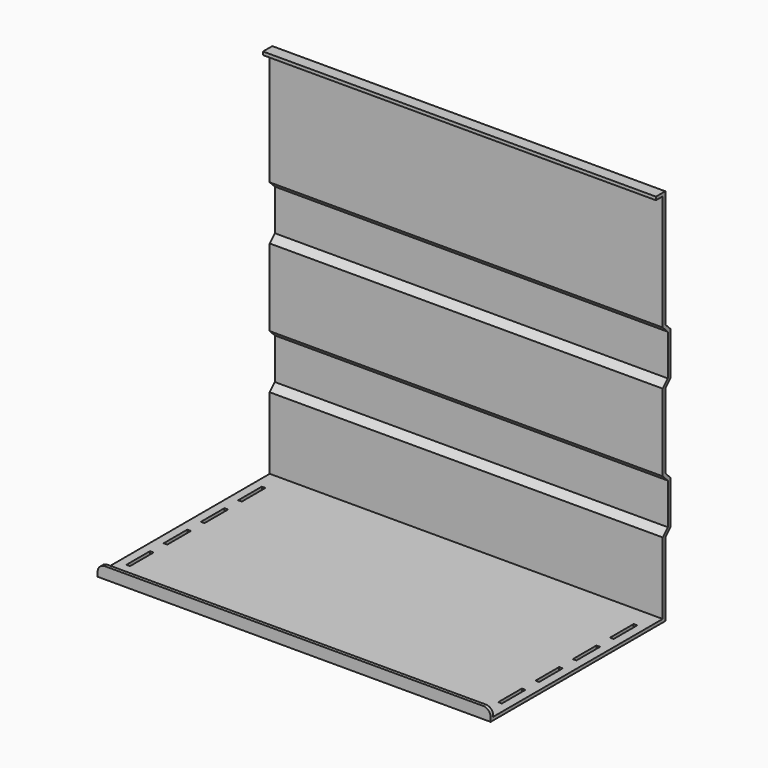
from build123d import *

# Parameters (mm, degrees)
F0_W     = 5.800000261
F0_H     = 2.2
F0_W_2   = 2.2
F0_H_2   = 5.8
F1_DEPTH = 270
F2_R     = 5
F3_W     = 2.5
F3_H     = 20.3
F4_DEPTH = 25


with BuildPart() as f1:
    # F0 (on Right) → F1 (new body)
    with BuildSketch(Plane.YZ):
        Polygon((-14.3636103166, 75.9268823147), (-14.3636103166, 68.1268823147), (-14.3636103166, -0.2731176853), (-12.1636103166, -2.4731176853), (-12.1636103166, 68.1268823147), (-12.1636103166, 75.9268823147), align=None)
        Polygon((-12.1636103166, -2.4731176853), (-14.3636103166, -0.2731176853), (-14.3636103166, -3.3843875225), (-12.1636103166, -5.5843875225), align=None)
        with Locations((-17.2636104471, 77.0268823147)):
            Rectangle(F0_W, F0_H)
        with Locations((-13.2636103166, 77.0268823147)):
            Rectangle(F0_W_2, F0_H)
        Polygon((-7.7636103166, -6.8731176853), (-12.1636103166, -2.4731176853), (-12.1636103166, -5.5843875225), (-9.9636103166, -7.7843875225), (-9.9636103166, -35.9618478481), (-12.1636103166, -38.1618478481), (-12.1636103166, -41.2731176853), (-7.7636103166, -36.8731176853), align=None)
        Polygon((-14.3636103166, -43.4731176853), (-12.1636103166, -41.2731176853), (-12.1636103166, -38.1618478481), (-14.3636103166, -40.3618478481), align=None)
        Polygon((-12.1636103166, -92.4731176853), (-12.1636103166, -41.2731176853), (-14.3636103166, -43.4731176853), (-14.3636103166, -90.2731176853), align=None)
        Polygon((-7.7636103166, -96.8731176853), (-12.1636103166, -92.4731176853), (-12.1636103166, -95.5843875225), (-9.9636103166, -97.7843875225), (-9.9636103166, -125.9618478481), (-12.1636103166, -128.1618478481), (-12.1636103166, -131.2731176853), (-7.7636103166, -126.8731176853), align=None)
        Polygon((-12.1636103166, -95.5843875225), (-12.1636103166, -92.4731176853), (-14.3636103166, -90.2731176853), (-14.3636103166, -93.3843875225), align=None)
        Polygon((-14.3636103166, -133.4731176853), (-12.1636103166, -131.2731176853), (-12.1636103166, -128.1618478481), (-14.3636103166, -130.3618478481), align=None)
        Polygon((-12.1636103166, -179.6731176853), (-12.1636103166, -131.2731176853), (-14.3636103166, -133.4731176853), (-14.3636103166, -179.6731176853), align=None)
        Polygon((-12.1636103166, -181.8731176853), (-12.1636103166, -179.6731176853), (-14.3636103166, -179.6731176853), (-159.9636103166, -179.6731176853), (-159.9636103166, -181.8731176853), align=None)
        with Locations((-161.0636103166, -180.7731176853)):
            Rectangle(F0_W_2, F0_H)
        with Locations((-161.0636103166, -176.7731176853)):
            Rectangle(F0_W_2, F0_H_2)
    extrude(amount=F1_DEPTH)

    # F2
    f2_edges = [f1.edges().sort_by_distance(p)[0] for p in [
        (270, -161.06361, -173.873118),
        (0, -161.06361, -173.873118),
    ]]
    fillet(f2_edges, radius=F2_R)

    # F3 (on face) → F4 (cut)
    with BuildSketch(Plane.XY.offset(-179.6731176853)):
        with Locations((7.25, -134.8136103166)):
            Rectangle(F3_W, F3_H)
        with Locations((7.25, -102.8136103166)):
            Rectangle(F3_W, F3_H)
        with Locations((7.25, -70.8136103166)):
            Rectangle(F3_W, F3_H)
        with Locations((7.25, -38.8136103166)):
            Rectangle(F3_W, F3_H)
        with Locations((262.75, -134.8136103166)):
            Rectangle(F3_W, F3_H)
        with Locations((262.75, -102.8136103166)):
            Rectangle(F3_W, F3_H)
        with Locations((262.75, -70.8136103166)):
            Rectangle(F3_W, F3_H)
        with Locations((262.75, -38.8136103166)):
            Rectangle(F3_W, F3_H)
    extrude(amount=-F4_DEPTH, mode=Mode.SUBTRACT)


solid = f1.part
